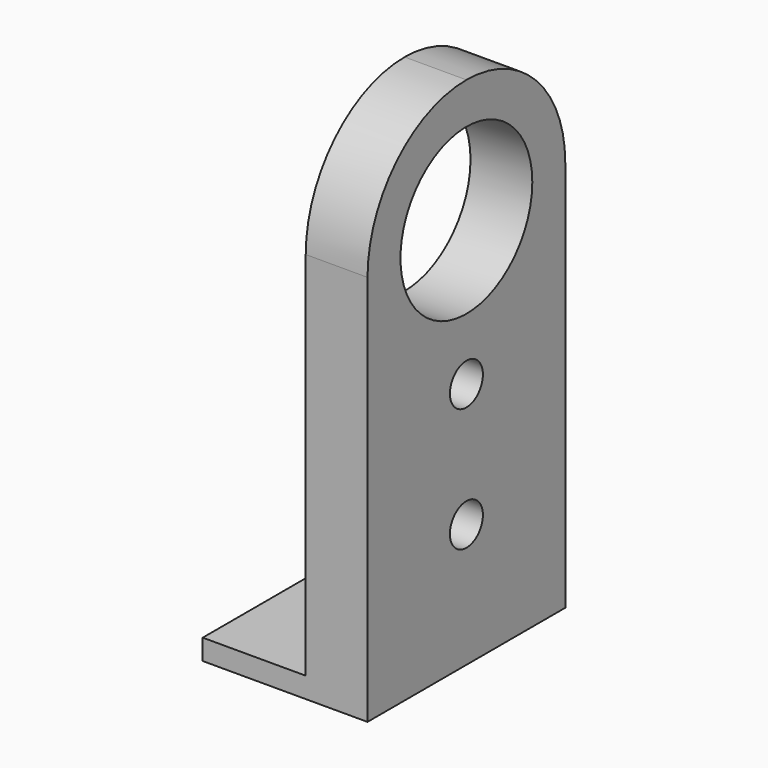
from build123d import *

# Parameters (mm, degrees)
F0_W     = 5
F0_H     = 12
F0_R     = 1
F1_DEPTH = 1
F0_W_2   = 3
F2_DEPTH = 25
F3_R     = 4
F3_R_2   = 1
F4_DEPTH = 3
F5_R     = 5.99999


# Not quite as in the source:
# - a fillet or chamfer is up to 0.001 mm smaller than in the source, because OpenCascade refuses the exact size


with BuildPart() as f1:
    # F0 (on Top) → F1 (new body)
    with BuildSketch(Plane.XY):
        with Locations((-14.9452780058, -4.4979301263)):
            Rectangle(F0_W, F0_H)
        with Locations((-14.9452780058, -4.4979301263)):
            Circle(F0_R, mode=Mode.SUBTRACT)
    extrude(amount=F1_DEPTH)

    # F0 (on Top) → F2 (join)
    with BuildSketch(Plane.XY):
        with Locations((-10.9452780058, -4.4979301263)):
            Rectangle(F0_W_2, F0_H)
    extrude(amount=F2_DEPTH)

    # F3 (on face) → F4 (cut)
    with BuildSketch(Plane.YZ.offset(-9.4452780058)):
        with Locations((-4.4979301263, 19)):
            Circle(F3_R)
        with Locations((-4.4979301263, 12)):
            Circle(F3_R_2)
        with Locations((-4.4979301263, 6)):
            Circle(F3_R_2)
    extrude(amount=-F4_DEPTH, mode=Mode.SUBTRACT)

    # F5 (radius 6 in the source; OpenCascade refuses exactly that, so slightly less here)
    f5_edges = [f1.edges().sort_by_distance(p)[0] for p in [
        (-10.945278, 1.50207, 25),
        (-10.945278, -10.49793, 25),
    ]]
    fillet(f5_edges, radius=F5_R)


solid = f1.part
